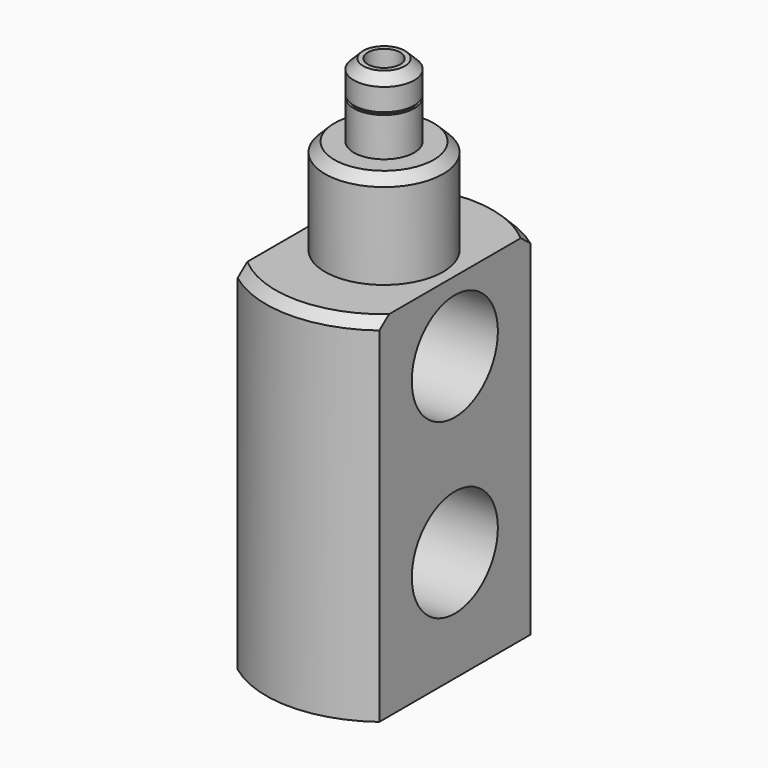
from build123d import *

# Parameters (mm, degrees)
F0_R      = 25.4
F1_DEPTH  = 76.2
F2_R      = 12.7124561547
F3_DEPTH  = 20.574
F4_R      = 6.5036133295
F5_DEPTH  = 8.382
F6_R      = 5.5261881266
F7_DEPTH  = 0.3556
F8_R      = 6.0681325209
F9_DEPTH  = 0.5588
F10_R     = 6.5080423993
F11_DEPTH = 6.8072
F12_W     = 12.8267863765
F12_H     = 46.3458411396
F13_DEPTH = 254
F14_W     = 15.4017303139
F14_H     = 51.6813602298
F15_DEPTH = 254
F16_R     = 11.58530812
F17_DEPTH = 254
F18_R     = 11.5775255265
F19_DEPTH = 254
F20_SIZE  = 2.032
F21_SIZE  = 2.032
F24_R     = 3.4812427805
F25_DEPTH = 50.8


# Not quite as in the source:
# - two fillets or chamfers of one size are made in one step


with BuildPart() as f1:
    # F0 (on Top) → F1 (new body)
    with BuildSketch(Plane.XY):
        Circle(F0_R)
    extrude(amount=F1_DEPTH)

    # F2 (on face) → F3 (join)
    with BuildSketch(Plane.XY.offset(76.2)):
        Circle(F2_R)
    extrude(amount=F3_DEPTH)

    # F4 (on face) → F5 (join)
    with BuildSketch(Plane.XY.offset(96.774)):
        Circle(F4_R)
    extrude(amount=F5_DEPTH)

    # F6 (on face) → F7 (join)
    with BuildSketch(Plane.XY.offset(105.156)):
        Circle(F6_R)
    extrude(amount=-F7_DEPTH)

    # F8 (on face) → F9 (join)
    with BuildSketch(Plane.XY.offset(105.156)):
        Circle(F8_R)
    extrude(amount=F9_DEPTH)

    # F10 (on face) → F11 (join)
    with BuildSketch(Plane.XY.offset(105.7148)):
        Circle(F10_R)
    extrude(amount=F11_DEPTH)

    # F12 (on face) → F13 (cut)
    with BuildSketch(Plane.XY.offset(76.2)):
        with Locations((-21.7024399899, -0.1023318619)):
            Rectangle(F12_W, F12_H)
    extrude(amount=-F13_DEPTH, mode=Mode.SUBTRACT)

    # F14 (on face) → F15 (cut)
    with BuildSketch(Plane.XY.offset(76.2)):
        with Locations((22.9368926957, -0.5596792325)):
            Rectangle(F14_W, F14_H)
    extrude(amount=-F15_DEPTH, mode=Mode.SUBTRACT)

    # F16 (on face) → F17 (cut)
    with BuildSketch(Plane.YZ.offset(15.2360275388)):
        with Locations((0, 61.0498785973)):
            Circle(F16_R)
    extrude(amount=-F17_DEPTH, mode=Mode.SUBTRACT)

    # F18 (on face) → F19 (cut)
    with BuildSketch(Plane.YZ.offset(15.2360275388)):
        with Locations((0, 23.8405317068)):
            Circle(F18_R)
    extrude(amount=-F19_DEPTH, mode=Mode.SUBTRACT)

    # F20
    f20_edges = [f1.edges().sort_by_distance(p)[0] for p in [
        (-0.033165, 25.399978, 76.2),
        (-0.033165, -25.399978, 76.2),
    ]]
    chamfer(f20_edges, length=F20_SIZE)

    # F21
    f21_edges = [f1.edges().sort_by_distance(p)[0] for p in [
        (-12.712456, 0, 96.774),
        (-6.508042, 0, 112.522),
    ]]
    chamfer(f21_edges, length=F21_SIZE)

    # F24 (on face) → F25 (cut)
    with BuildSketch(Plane.XY.offset(112.522)):
        Circle(F24_R)
    extrude(amount=-F25_DEPTH, mode=Mode.SUBTRACT)


solid = f1.part
